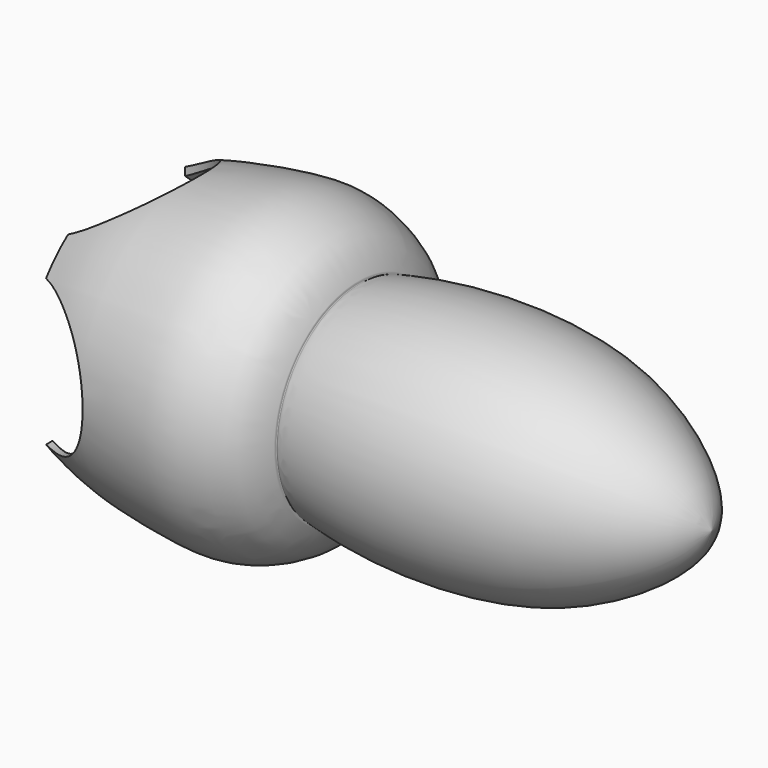
from build123d import *

# Parameters (mm, degrees)
F2_DEPTH      = 100
F2_DEPTH_BACK = 100
F4_DEPTH      = 100
F4_DEPTH_BACK = 100


with BuildPart() as f1:
    # F0 (on Front) → F1 (revolve)
    with BuildSketch(Plane.XZ):
        with BuildLine():
            add(Edge.make_bspline(
                [(-90.8851660788, -36.2573902607), (-88.5852130802, -37.2254113047), (-83.5024287867, -39.3419551547), (-73.4407189284, -42.6576256114), (-49.4695844523, -46.6517874504), (-37.8265257132, -45.647753558), (-24.526945208, -39.2846355217), (-21.9079329007, -32.8877596775), (-20.544440952, -30.8136017692), (-20.2924121124, -29.6541500081), (-19.0985399903, -30.1130116783), (-17.3486522149, -30.7160657532), (-2.3869854339, -33.1511866039), (18.59878364, -35.0645887105), (48.4681184214, -30.9731938746), (62.8312124415, -23.0672274533), (82.6724215491, -10.9698241493), (85.7379966236, -3.2524782478), (86.8547097914, -0.8886294858), (87.1148339212, 0)],
                knots=[0, 0, 0, 0, 0.0520597762, 0.1146371802, 0.2071341803, 0.2742100064, 0.3443736144, 0.3926207753, 0.4215586148, 0.4390558705, 0.457107598, 0.4817305795, 0.5518061066, 0.6428901289, 0.7447591917, 0.8241971476, 0.9135763965, 0.9662130015, 1, 1, 1, 1], degree=3))
            add(Edge.make_bspline(
                [(-90.8851660788, -36.2573902607), (-90.8851660788, -36.9240569274), (-90.8851660788, -37.590723594), (-90.8851660788, -38.2573902607)],
                knots=[36.2573902607, 36.2573902607, 36.2573902607, 36.2573902607, 38.2573902607, 38.2573902607, 38.2573902607, 38.2573902607], degree=3))
            add(Edge.make_bspline(
                [(89.1148339212, 0), (87.9535407963, -3.4927117631), (84.6721152508, -13.2460658398), (49.1761477479, -37.0431155105), (-1.0985229918, -36.123394382), (-18.2811955687, -32.0566776123), (-18.9010085353, -32.0074722013), (-19.5975226606, -31.3497657837), (-19.4094320071, -32.2760287195), (-19.9762208078, -32.9917027018), (-22.8020885815, -41.0650686213), (-37.1643063714, -47.4967821273), (-49.724112546, -48.3304066252), (-73.7538573246, -44.3413675223), (-83.946030413, -40.9934318301), (-88.750846708, -39.0989379622), (-90.8851660788, -38.2573902607)],
                knots=[0, 0, 0, 0, 0.0776921241, 0.2183842806, 0.3798351112, 0.4637230565, 0.4790803126, 0.4959506909, 0.5120411522, 0.5321494253, 0.5925027077, 0.6782407003, 0.7593910583, 0.8679142282, 0.9413056264, 1, 1, 1, 1], degree=3))
            Line((89.1148339212, 0), (87.1148339212, 0))
        make_face()
    revolve(axis=Axis((-51.1527098715, 0, 0), (-1, 0, 0)))

    # F0 (on Front) → F2 (cut, two sides)
    with BuildSketch(Plane.XZ) as f2_sk:
        with BuildLine():
            add(Edge.make_bspline(
                [(-90.8851660788, 0), (-90.8851660788, -7.5), (-90.8851660788, -15), (-90.8851660788, -22.5)],
                knots=[0, 0, 0, 0, 22.5, 22.5, 22.5, 22.5], degree=3))
            Line((-90.8851660788, 0), (-68.3851660788, 0))
            ThreePointArc((-68.3851660788, 0), (-106.7950686555, 15.9099025767), (-90.8851660788, -22.5))
        make_face()
        with BuildLine():
            Line((-68.3851660788, 0), (-90.8851660788, 0))
            add(Edge.make_bspline(
                [(-90.8851660788, 0), (-90.8851660788, -7.5), (-90.8851660788, -15), (-90.8851660788, -22.5)],
                knots=[0, 0, 0, 0, 22.5, 22.5, 22.5, 22.5], degree=3))
            ThreePointArc((-90.8851660788, -22.5), (-74.9752635021, -15.9099025767), (-68.3851660788, 0))
        make_face()
    extrude(amount=-F2_DEPTH, mode=Mode.SUBTRACT)
    extrude(f2_sk.sketch, amount=F2_DEPTH_BACK, mode=Mode.SUBTRACT)

    # F3 (on Top) → F4 (cut, two sides)
    with BuildSketch(Plane.XY) as f4_sk:
        with BuildLine():
            ThreePointArc((-90.8851660788, 22.5), (-113.3851660788, 0), (-90.8851660788, -22.5))
            Line((-90.8851660788, -22.5), (-90.8851660788, 22.5))
        make_face()
        with BuildLine():
            Line((-90.8851660788, 22.5), (-90.8851660788, -22.5))
            ThreePointArc((-90.8851660788, -22.5), (-74.9752635021, -15.9099025767), (-68.3851660788, 0))
            ThreePointArc((-68.3851660788, 0), (-74.9752635021, 15.9099025767), (-90.8851660788, 22.5))
        make_face()
    extrude(amount=-F4_DEPTH, mode=Mode.SUBTRACT)
    extrude(f4_sk.sketch, amount=F4_DEPTH_BACK, mode=Mode.SUBTRACT)


solid = f1.part
